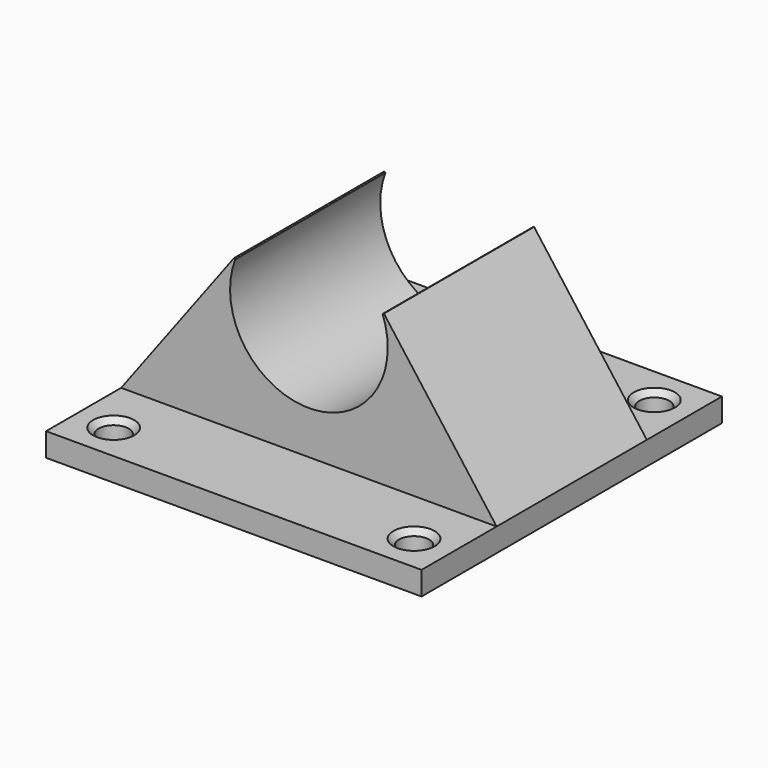
from build123d import *

# Parameters (mm, degrees)
F0_W        = 50.8
F0_H        = 50.8
F1_DEPTH    = 3.175
F3_DEPTH    = 12.7
F4_T1_DEPTH = 29.6642315955
F5_R        = 2.032
F6_DEPTH    = 25.4
F7_SIZE     = 0.762


# Not quite as in the source:
# - a fillet or chamfer that OpenCascade refuses, or shapes differently, is made with other operations: its cross-section is extruded or revolved along the edge and cut away or added


with BuildPart() as f1:
    # F0 (on Top) → F1 (new body)
    with BuildSketch(Plane.XY):
        Rectangle(F0_W, F0_H)
    extrude(amount=F1_DEPTH)

    # F2 (on Front) → F3 (join, symmetric)
    with BuildSketch(Plane.XZ):
        with BuildLine():
            ThreePointArc((9.6386223082, 24.257), (0, 9.017), (-9.6386223082, 24.257))
            Line((-9.6386223082, 24.257), (-25.4, 3.175))
            Line((-25.4, 3.175), (25.4, 3.175))
            Line((25.4, 3.175), (9.6386223082, 24.257))
        make_face()
    extrude(amount=F3_DEPTH, both=True)

    # F4: chamfer of 1.016 on 2 edges, made by hand

    # F4_s2 → F4_t1 (cut)
    with BuildSketch(Plane.XZ.offset(-14.8321157977)):
        with BuildLine():
            Line((-10.1809562751, 23.5988049587), (-9.9336646357, 23.4627576649))
            Line((-9.9336646357, 23.4627576649), (-9.9146755466, 23.4555246232))
            ThreePointArc((-9.9146755466, 23.4555246232), (-9.7936995215, 23.8631023282), (-9.6202630276, 24.2482914286))
            Line((-9.6202630276, 24.2482914286), (-9.6548968618, 24.2691672226))
            ThreePointArc((-9.6548968618, 24.2691672226), (-9.9099463042, 23.9280198655), (-10.1972308287, 23.6109721813))
            Line((-10.1972308287, 23.6109721813), (-10.1809562751, 23.5988049587))
        make_face()
        with BuildLine():
            Line((10.1809562751, 23.5988049587), (9.9336646357, 23.4627576649))
            Line((9.9336646357, 23.4627576649), (9.9146755466, 23.4555246232))
            ThreePointArc((9.9146755466, 23.4555246232), (9.7936995215, 23.8631023282), (9.6202630276, 24.2482914286))
            Line((9.6202630276, 24.2482914286), (9.6548968618, 24.2691672226))
            ThreePointArc((9.6548968618, 24.2691672226), (9.9099463042, 23.9280198655), (10.1972308287, 23.6109721813))
            Line((10.1972308287, 23.6109721813), (10.1809562751, 23.5988049587))
        make_face()
    extrude(amount=F4_T1_DEPTH, mode=Mode.SUBTRACT)

    # F5 (on face) → F6 (cut)
    with BuildSketch(Plane(origin=(0, 0, 0), x_dir=(1, 0, 0), z_dir=(0, 0, -1))):
        with Locations((-20.32, 20.32)):
            Circle(F5_R)
        with Locations((-20.32, -20.32)):
            Circle(F5_R)
        with Locations((20.32, 20.32)):
            Circle(F5_R)
        with Locations((20.32, -20.32)):
            Circle(F5_R)
    extrude(amount=-F6_DEPTH, mode=Mode.SUBTRACT)

    # F7
    f7_edges = [f1.edges().sort_by_distance(p)[0] for p in [
        (-22.352, -20.32, 3.175),
        (-22.352, 20.32, 3.175),
        (18.288, 20.32, 3.175),
        (18.288, -20.32, 3.175),
    ]]
    chamfer(f7_edges, length=F7_SIZE)


solid = f1.part
